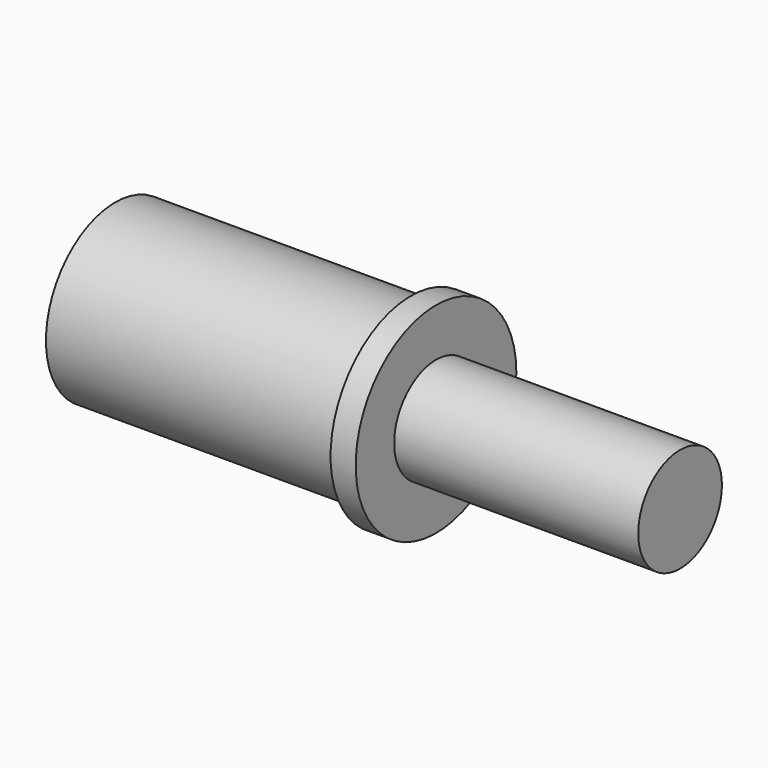
from build123d import *

# Parameters (mm, degrees)
F0_R     = 7.8867
F1_DEPTH = 26.924
F0_R_2   = 9.144
F2_DEPTH = 2.286
F3_R     = 4.7625
F4_DEPTH = 22.225


# Not quite as in the source:
# - a length typed as a fraction of an inch, garbled in the dataset ("3 / 203.2 mm" for 3/8 in), is restored


with BuildPart() as f1:
    # F0 (on Right) → F1 (new body)
    with BuildSketch(Plane.YZ):
        Circle(F0_R)
    extrude(amount=-F1_DEPTH)

    # F0 (on Right) → F2 (join)
    with BuildSketch(Plane.YZ):
        Circle(F0_R_2)
        Circle(F0_R, mode=Mode.SUBTRACT)
        Circle(F0_R)
    extrude(amount=F2_DEPTH)

    # F3 (on face) → F4 (join)
    with BuildSketch(Plane.YZ.offset(2.286)):
        Circle(F3_R)
    extrude(amount=F4_DEPTH)


solid = f1.part
